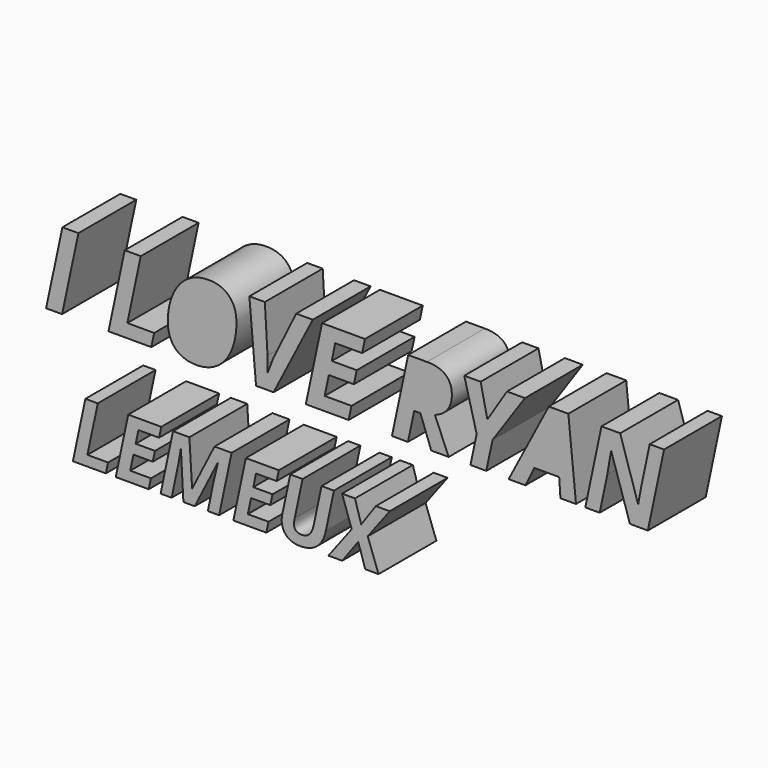
from build123d import *

# Parameters (mm, degrees)
F0_TEXT_SIZE   = 37.7067726933
F0_TEXT_SIZE_2 = 29.0437077638
F1_DEPTH       = 25.4


# Not quite as in the source:
# - Text() gives the source's letters only with a copy of the font that has no kerning and outlines rounded to 1/6400 em; it was checked with that copy


with BuildPart() as f1:
    # F0 (on Front) → F1 (new body)
    with BuildSketch(Plane.XZ):
        with BuildLine():
            add(Edge.make_bspline(
                [(-27.3255350451, 59.7530705402), (-28.5215467415, 61.1788578826), (-30.6955778546, 61.1788578826)],
                knots=[0, 0, 0, 1, 1, 1], degree=2))
            add(Edge.make_bspline(
                [(-30.6955778546, 61.1788578826), (-32.9226341168, 61.1788578826), (-34.7814601769, 59.4967823195)],
                knots=[0, 0, 0, 1, 1, 1], degree=2))
            add(Edge.make_bspline(
                [(-34.7814601769, 59.4967823195), (-36.640286237, 57.8147067564), (-37.700789219, 54.8688651397)],
                knots=[0, 0, 0, 1, 1, 1], degree=2))
            add(Edge.make_bspline(
                [(-37.700789219, 54.8688651397), (-38.761292201, 51.9230235231), (-38.761292201, 48.4763888316)],
                knots=[0, 0, 0, 1, 1, 1], degree=2))
            add(Edge.make_bspline(
                [(-38.761292201, 48.4763888316), (-38.761292201, 45.7721062275), (-37.5358220885, 44.3905065092)],
                knots=[0, 0, 0, 1, 1, 1], degree=2))
            add(Edge.make_bspline(
                [(-37.5358220885, 44.3905065092), (-36.310351976, 43.008906791), (-34.0832957138, 43.008906791)],
                knots=[0, 0, 0, 1, 1, 1], degree=2))
            add(Edge.make_bspline(
                [(-34.0832957138, 43.008906791), (-31.8562394516, 43.008906791), (-30.023925966, 44.6114446305)],
                knots=[0, 0, 0, 1, 1, 1], degree=2))
            add(Edge.make_bspline(
                [(-30.023925966, 44.6114446305), (-28.1916124804, 46.21398247), (-27.1605679146, 49.1421490369)],
                knots=[0, 0, 0, 1, 1, 1], degree=2))
            add(Edge.make_bspline(
                [(-27.1605679146, 49.1421490369), (-26.1295233488, 52.0703156039), (-26.1295233488, 55.7113758421)],
                knots=[0, 0, 0, 1, 1, 1], degree=2))
            add(Edge.make_bspline(
                [(-26.1295233488, 55.7113758421), (-26.1295233488, 58.3272831977), (-27.3255350451, 59.7530705402)],
                knots=[0, 0, 0, 1, 1, 1], degree=2))
        make_face()
        with Locations((-88.2160812616, 38.590144366)):
            Text('I LOVE RYAN', F0_TEXT_SIZE, font='Open Sans', font_style=FontStyle.BOLDITALIC, text_align=(TextAlign.LEFT, TextAlign.BOTTOM))
        with Locations((-78.5695835948, -5.6468206458)):
            Text('LEMEUX', F0_TEXT_SIZE_2, font='Open Sans', font_style=FontStyle.BOLDITALIC, text_align=(TextAlign.LEFT, TextAlign.BOTTOM))
        with BuildLine():
            Line((44.5588920848, 60.8312485719), (43.0093793944, 53.5609114619))
            Line((43.0093793944, 53.5609114619), (44.4469501033, 53.5609114619))
            add(Edge.make_bspline(
                [(44.4469501033, 53.5609114619), (46.8566485458, 53.5609114619), (48.2028981646, 54.6096310775)],
                knots=[0, 0, 0, 1, 1, 1], degree=2))
            add(Edge.make_bspline(
                [(48.2028981646, 54.6096310775), (49.5491477834, 55.658350693), (49.5491477834, 57.8147067564)],
                knots=[0, 0, 0, 1, 1, 1], degree=2))
            add(Edge.make_bspline(
                [(49.5491477834, 57.8147067564), (49.5491477834, 59.3229776641), (48.6742328232, 60.077113118)],
                knots=[0, 0, 0, 1, 1, 1], degree=2))
            add(Edge.make_bspline(
                [(48.6742328232, 60.077113118), (47.7993178631, 60.8312485719), (45.9198709117, 60.8312485719)],
                knots=[0, 0, 0, 1, 1, 1], degree=2))
            Line((45.9198709117, 60.8312485719), (44.5588920848, 60.8312485719))
        make_face()
        with BuildLine():
            Line((86.5724852216, 49.7843425094), (92.6998357843, 49.7843425094))
            Line((92.6998357843, 49.7843425094), (92.2226094424, 56.2298439666))
            add(Edge.make_bspline(
                [(92.2226094424, 56.2298439666), (92.0399672622, 58.6395424091), (92.0399672622, 60.884273721)],
                knots=[0, 0, 0, 1, 1, 1], degree=2))
            Line((92.0399672622, 60.884273721), (92.0399672622, 61.5500339263))
            add(Edge.make_bspline(
                [(92.0399672622, 61.5500339263), (91.226914976, 59.3406527138), (90.0309032796, 56.8720374391)],
                knots=[0, 0, 0, 1, 1, 1], degree=2))
            Line((90.0309032796, 56.8720374391), (86.5724852216, 49.7843425094))
        make_face()
    extrude(amount=F1_DEPTH)


solid = f1.part
